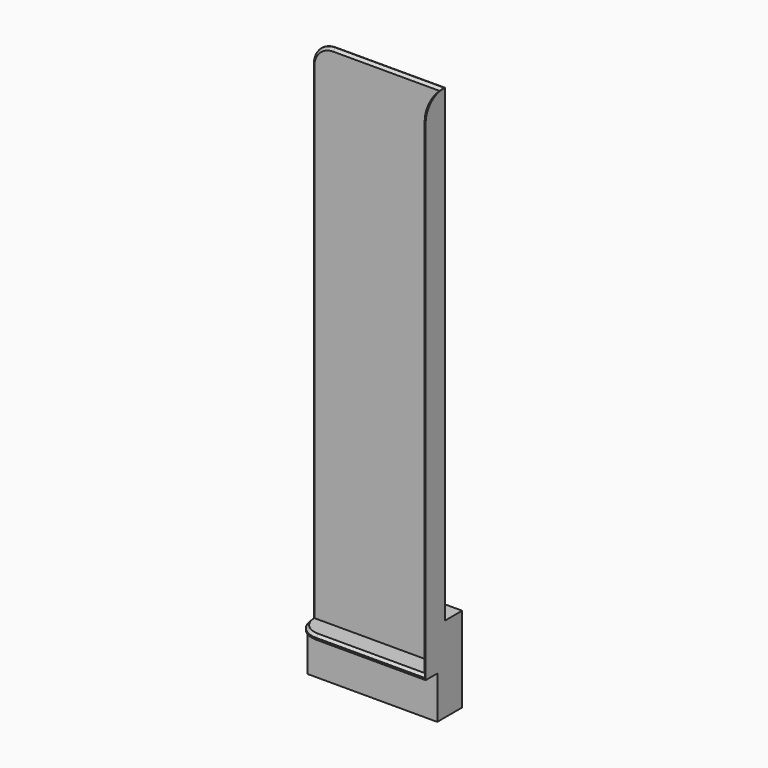
from build123d import *

# Parameters (mm, degrees)
F0_W      = 76.2
F0_H      = 304.8
F1_DEPTH  = 1.778
F2_W      = 76.2
F2_H      = 2.54
F3_DEPTH  = 12.7
F4_W      = 14.478
F4_H      = 304.8
F5_DEPTH  = 1.778
F4_W_2    = 0.1264255261
F4_H_2    = 0.0905882334
F6_W      = 77.978
F6_H      = 5.842
F7_DEPTH  = 25.4
F8_W      = 52.324
F8_H      = 50.8
F9_DEPTH  = 10.16
F11_W     = 52.832
F11_H     = 50.8
F12_DEPTH = 12.7
F13_R     = 12.7
F14_R     = 12.7
F15_R     = 12.7
F16_SIZE  = 1.524
F17_SIZE  = 1.523


# Not quite as in the source:
# - a fillet or chamfer is up to 0.001 mm smaller than in the source, because OpenCascade refuses the exact size


with BuildPart() as f1:
    # F0 (on Front) → F1 (new body)
    with BuildSketch(Plane.XZ):
        with Locations((38.1, 152.4)):
            Rectangle(F0_W, F0_H)
    extrude(amount=F1_DEPTH)

    # F2 (on face) → F3 (join)
    with BuildSketch(Plane.XZ.offset(1.778)):
        with Locations((38.1, 1.27)):
            Rectangle(F2_W, F2_H)
    extrude(amount=F3_DEPTH)

    # F4 (on face) → F5 (join)
    with BuildSketch(Plane.YZ.offset(76.2)):
        with Locations((-7.239, 152.4)):
            Rectangle(F4_W, F4_H)
    extrude(amount=F5_DEPTH)

    # F6 (on face) → F7 (join)
    with BuildSketch(Plane(origin=(0, 0, 0), x_dir=(1, 0, 0), z_dir=(0, 0, -1))):
        with Locations((38.989, 2.921)):
            Rectangle(F6_W, F6_H)
    extrude(amount=F7_DEPTH)

    # F11 (on face) → F12 (join)
    with BuildSketch(Plane(origin=(0, 0, 0), x_dir=(-1, 0, 0), z_dir=(0, 1, 0))):
        with Locations((-51.562, 0)):
            Rectangle(F11_W, F11_H)
    extrude(amount=F12_DEPTH)

    # F13
    f13_edges = [f1.edges().sort_by_distance(p)[0] for p in [
        (0, -0.889, 304.8),
    ]]
    fillet(f13_edges, radius=F13_R)

    # F14
    f14_edges = [f1.edges().sort_by_distance(p)[0] for p in [
        (77.089, -14.478, 304.8),
    ]]
    fillet(f14_edges, radius=F14_R)

    # F15
    f15_edges = [f1.edges().sort_by_distance(p)[0] for p in [
        (0, -14.478, 1.27),
    ]]
    fillet(f15_edges, radius=F15_R)

    # F16
    f16_edges = [f1.edges().sort_by_distance(p)[0] for p in [
        (0, -1.778, 147.32),
    ]]
    chamfer(f16_edges, length=F16_SIZE)

    # F17 (size 1.524 in the source; OpenCascade refuses exactly that, so slightly less here)
    f17_edges = [f1.edges().sort_by_distance(p)[0] for p in [
        (3.719744, -10.758256, 2.54),
        (44.45, -14.478, 2.54),
        (76.2, -14.478, 147.32),
    ]]
    chamfer(f17_edges, length=F17_SIZE)


with BuildPart() as f5:
    # F4 (on face) → F5, piece 2 (new body)
    with BuildSketch(Plane.YZ.offset(76.2)):
        with Locations((1.1594051612, 0.5721470225)):
            Rectangle(F4_W_2, F4_H_2)
    extrude(amount=F5_DEPTH)


with BuildPart() as f9:
    # F8 (on face) → F9 (new body)
    with BuildSketch(Plane(origin=(0, 0, 0), x_dir=(-1, 0, 0), z_dir=(0, 1, 0))):
        with Locations((-51.816, 0)):
            Rectangle(F8_W, F8_H)
    extrude(amount=F9_DEPTH)


solid = f1.part
